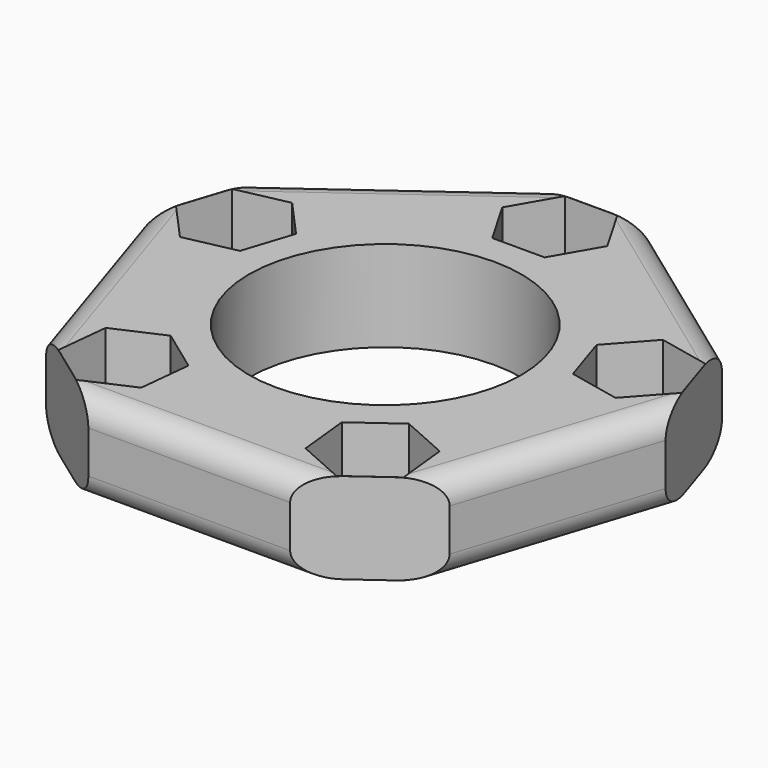
from build123d import *

# Parameters (mm, degrees)
F0_R        = 14.2875
F1_DEPTH    = 9.525
F2_SIZE     = 8.0772
F3_T1_DEPTH = 33.8699635206
F3_T3_DEPTH = 33.8699635206
F3_T5_DEPTH = 33.8699635206
F3_T7_DEPTH = 33.8699635206
F3_T9_DEPTH = 33.8699635206
F4_T1_DEPTH = 33.8699635206
F4_T3_DEPTH = 33.8699635206
F4_T5_DEPTH = 33.8699635206
F4_T7_DEPTH = 33.8699635206
F4_T9_DEPTH = 33.8699635206


# Not quite as in the source:
# - a fillet or chamfer that OpenCascade refuses, or shapes differently, is made with other operations: its cross-section is extruded or revolved along the edge and cut away or added


with BuildPart() as f1:
    # F0 (on Top) → F1 (new body)
    with BuildSketch(Plane.XY):
        Polygon((30.1960443924, 9.8112895714), (0, 31.75), (-30.1960443924, 9.8112895714), (-18.6621817603, -25.6862895714), (18.6621817603, -25.6862895714), align=None)
        Polygon((-18.087352426, -20.2171537862), (-17.5125230918, -14.7480180011), (-12.4886978979, -12.5112669148), (-8.0397020384, -15.7436516137), (-8.6145313726, -21.2127873989), (-13.6383565665, -23.4495384851), align=None, mode=Mode.SUBTRACT)
        Circle(F0_R, mode=Mode.SUBTRACT)
        Polygon((13.6383565665, -23.4495384851), (8.6145313726, -21.2127873989), (8.0397020384, -15.7436516137), (12.4886978979, -12.5112669148), (17.5125230918, -14.7480180011), (18.087352426, -20.2171537862), align=None, mode=Mode.SUBTRACT)
        Polygon((-24.8169551322, 10.9546502895), (-19.4378658721, 12.0980110075), (-15.7581418145, 8.011263418), (-17.4575070171, 2.7811551105), (-22.8365962772, 1.6377943925), (-26.5163203348, 5.7245419819), align=None, mode=Mode.SUBTRACT)
        Polygon((-5.499261314, 22.225), (-2.749630657, 26.9875), (2.749630657, 26.9875), (5.499261314, 22.225), (2.749630657, 17.4625), (-2.749630657, 17.4625), align=None, mode=Mode.SUBTRACT)
        Polygon((26.5163203348, 5.7245419819), (22.8365962772, 1.6377943925), (17.4575070171, 2.7811551105), (15.7581418145, 8.011263418), (19.4378658721, 12.0980110075), (24.8169551322, 10.9546502895), align=None, mode=Mode.SUBTRACT)
    extrude(amount=F1_DEPTH)

    # F2
    f2_edges = [f1.edges().sort_by_distance(p)[0] for p in [
        (-18.662182, -25.68629, 4.7625),
        (18.662182, -25.68629, 4.7625),
        (30.196044, 9.81129, 4.7625),
        (0, 31.75, 4.7625),
        (-30.196044, 9.81129, 4.7625),
    ]]
    chamfer(f2_edges, length=F2_SIZE)

    # F3: fillet of radius 2.54 on 5 edges, made by hand

    # F3_s2 → F3_t1 (cut)
    with BuildSketch(Plane(origin=(-5.2331971634, -16.1061247565, 0), x_dir=(0, 0, 1), z_dir=(0.3090169944, 0.9510565163, 0))):
        with BuildLine():
            ThreePointArc((9.525, 23.1462895714), (8.7810512242, 24.9423407956), (6.985, 25.6862895714))
            Line((6.985, 25.6862895714), (9.525, 25.6862895714))
            Line((9.525, 25.6862895714), (9.525, 23.1462895714))
        make_face()
    extrude(amount=F3_T1_DEPTH, mode=Mode.SUBTRACT)

    # F3_s4 → F3_t3 (cut)
    with BuildSketch(Plane.YZ.offset(-16.9349817603)):
        with BuildLine():
            ThreePointArc((-23.1462895714, 9.525), (-24.9423407956, 8.7810512242), (-25.6862895714, 6.985))
            Line((-25.6862895714, 6.985), (-25.6862895714, 9.525))
            Line((-25.6862895714, 9.525), (-23.1462895714, 9.525))
        make_face()
    extrude(amount=F3_T3_DEPTH, mode=Mode.SUBTRACT)

    # F3_s6 → F3_t5 (cut)
    with BuildSketch(Plane(origin=(-5.2331971634, 16.1061247565, 0), x_dir=(0, 0, 1), z_dir=(0.3090169944, -0.9510565163, 0))):
        with BuildLine():
            ThreePointArc((9.525, 23.1462895714), (8.7810512242, 24.9423407956), (6.985, 25.6862895714))
            Line((6.985, 25.6862895714), (9.525, 25.6862895714))
            Line((9.525, 25.6862895714), (9.525, 23.1462895714))
        make_face()
    extrude(amount=F3_T5_DEPTH, mode=Mode.SUBTRACT)

    # F3_s8 → F3_t7 (cut)
    with BuildSketch(Plane(origin=(13.7006880435, 9.9541325265, 0), x_dir=(0, 0, 1), z_dir=(-0.8090169944, -0.5877852523, 0))):
        with BuildLine():
            ThreePointArc((9.525, 23.1462895714), (8.7810512242, 24.9423407956), (6.985, 25.6862895714))
            Line((6.985, 25.6862895714), (9.525, 25.6862895714))
            Line((9.525, 25.6862895714), (9.525, 23.1462895714))
        make_face()
    extrude(amount=F3_T7_DEPTH, mode=Mode.SUBTRACT)

    # F3_s10 → F3_t9 (cut)
    with BuildSketch(Plane(origin=(13.7006880435, -9.9541325265, 0), x_dir=(0, 0, 1), z_dir=(-0.8090169944, 0.5877852523, 0))):
        with BuildLine():
            ThreePointArc((6.985, 25.6862895714), (8.7810512242, 24.9423407956), (9.525, 23.1462895714))
            Line((9.525, 23.1462895714), (9.525, 25.6862895714))
            Line((9.525, 25.6862895714), (6.985, 25.6862895714))
        make_face()
    extrude(amount=F3_T9_DEPTH, mode=Mode.SUBTRACT)

    # F4: fillet of radius 2.54 on 5 edges, made by hand

    # F4_s2 → F4_t1 (cut)
    with BuildSketch(Plane(origin=(-5.2331971634, -16.1061247565, 0), x_dir=(0, 0, 1), z_dir=(0.3090169944, 0.9510565163, 0))):
        with BuildLine():
            ThreePointArc((0, 23.1462895714), (0.7439487758, 24.9423407956), (2.54, 25.6862895714))
            Line((2.54, 25.6862895714), (0, 25.6862895714))
            Line((0, 25.6862895714), (0, 23.1462895714))
        make_face()
    extrude(amount=F4_T1_DEPTH, mode=Mode.SUBTRACT)

    # F4_s4 → F4_t3 (cut)
    with BuildSketch(Plane.YZ.offset(-16.9349817603)):
        with BuildLine():
            ThreePointArc((-23.1462895714, 0), (-24.9423407956, 0.7439487758), (-25.6862895714, 2.54))
            Line((-25.6862895714, 2.54), (-25.6862895714, 0))
            Line((-25.6862895714, 0), (-23.1462895714, 0))
        make_face()
    extrude(amount=F4_T3_DEPTH, mode=Mode.SUBTRACT)

    # F4_s6 → F4_t5 (cut)
    with BuildSketch(Plane(origin=(13.7006880435, 9.9541325265, 0), x_dir=(0, 0, 1), z_dir=(-0.8090169944, -0.5877852523, 0))):
        with BuildLine():
            ThreePointArc((0, 23.1462895714), (0.7439487758, 24.9423407956), (2.54, 25.6862895714))
            Line((2.54, 25.6862895714), (0, 25.6862895714))
            Line((0, 25.6862895714), (0, 23.1462895714))
        make_face()
    extrude(amount=F4_T5_DEPTH, mode=Mode.SUBTRACT)

    # F4_s8 → F4_t7 (cut)
    with BuildSketch(Plane(origin=(13.7006880435, -9.9541325265, 0), x_dir=(0, 0, 1), z_dir=(-0.8090169944, 0.5877852523, 0))):
        with BuildLine():
            ThreePointArc((2.54, 25.6862895714), (0.7439487758, 24.9423407956), (0, 23.1462895714))
            Line((0, 23.1462895714), (0, 25.6862895714))
            Line((0, 25.6862895714), (2.54, 25.6862895714))
        make_face()
    extrude(amount=F4_T7_DEPTH, mode=Mode.SUBTRACT)

    # F4_s10 → F4_t9 (cut)
    with BuildSketch(Plane(origin=(-5.2331971634, 16.1061247565, 0), x_dir=(0, 0, 1), z_dir=(0.3090169944, -0.9510565163, 0))):
        with BuildLine():
            ThreePointArc((0, 23.1462895714), (0.7439487758, 24.9423407956), (2.54, 25.6862895714))
            Line((2.54, 25.6862895714), (0, 25.6862895714))
            Line((0, 25.6862895714), (0, 23.1462895714))
        make_face()
    extrude(amount=F4_T9_DEPTH, mode=Mode.SUBTRACT)


solid = f1.part
